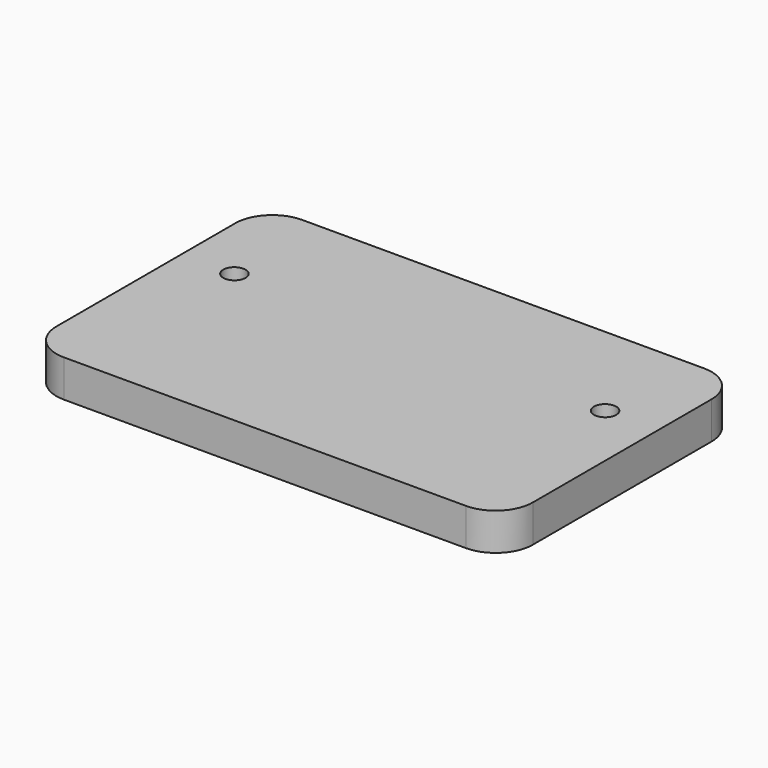
from build123d import *

# Parameters (mm, degrees)
F0_W     = 64
F0_H     = 40
F0_R     = 1.5
F1_DEPTH = 5
F2_R     = 5


# Not quite as in the source:
# - a feature names something its author has since deleted; it is built from what else it names


with BuildPart() as f1:
    # F0 (on Top) → F1 (new body)
    with BuildSketch(Plane.XY):
        with Locations((0, -35.9806431703)):
            Rectangle(F0_W, F0_H)
        with Locations((-24.9, -29.9806431703)):
            Circle(F0_R, mode=Mode.SUBTRACT)
        with Locations((24.9, -29.9806431703)):
            Circle(F0_R, mode=Mode.SUBTRACT)
    extrude(amount=F1_DEPTH)

    # F2
    f2_edges = [f1.edges().sort_by_distance(p)[0] for p in [
        (-32, -55.980643, 2.5),
        (32, -55.980643, 2.5),
        (32, -15.980643, 2.5),
        (-32, -15.980643, 2.5),
    ]]
    fillet(f2_edges, radius=F2_R)


solid = f1.part
